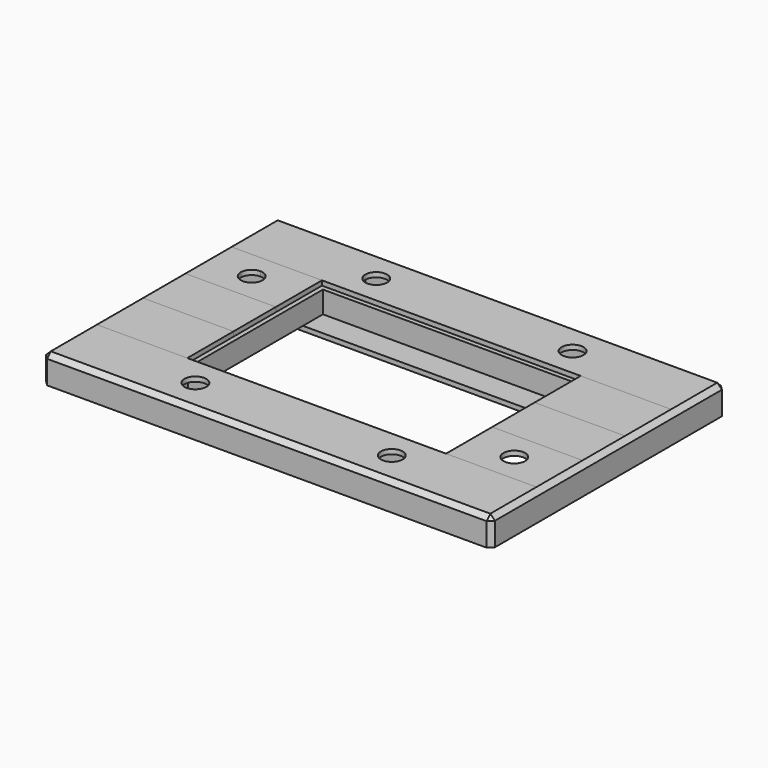
from build123d import *

# Parameters (mm, degrees)
F0_W       = 38.1
F0_H       = 38.1
F0_W_2     = 1016
F0_H_2     = 647.7
F0_W_3     = 311.15
F0_H_3     = 177.8
F1_DEPTH   = 88.9
F2_W       = 311.15
F2_H       = 177.8
F2_W_2     = 1016
F3_DEPTH   = 19.05
F2_H_2     = 215.9
F2_W_3     = 38.1
F2_W_4     = 19.05
F4_DEPTH   = 19.05
F5_W       = 1092.2
F5_H       = 139.7
F6_DEPTH   = 19.05
F7_W       = 1790.7
F7_H       = 114.3
F8_DEPTH   = 19.05
F9_W       = 1790.7
F9_H       = 114.3
F10_DEPTH  = 19.05
F11_W      = 1193.8
F11_H      = 114.3
F12_DEPTH  = 19.05
F13_W      = 1193.8
F13_H      = 114.3
F14_DEPTH  = 19.05
F15_SIZE   = 19.04999
F15_2_SIZE = 19.04999
F15_3_SIZE = 19.04999
F15_4_SIZE = 19.04999
F16_R      = 44.45
F17_DEPTH  = 19.05


# Not quite as in the source:
# - a fillet or chamfer is up to 0.001 mm smaller than in the source, because OpenCascade refuses the exact size


with BuildPart() as f1:
    # F0 (on Top) → F1 (new body)
    with BuildSketch(Plane.XY):
        with Locations((527.05, 558.8)):
            Rectangle(F0_W, F0_H)
        with Locations((0, 558.8)):
            Rectangle(F0_W_2, F0_H)
        with Locations((876.3, 0)):
            Rectangle(F0_W, F0_H_2)
        with Locations((876.3, 342.9)):
            Rectangle(F0_W, F0_H)
        with Locations((-876.3, 342.9)):
            Rectangle(F0_W, F0_H)
        with Locations((-876.3, 0)):
            Rectangle(F0_W, F0_H_2)
        with Locations((-527.05, 558.8)):
            Rectangle(F0_W, F0_H)
        with Locations((0, -558.8)):
            Rectangle(F0_W_2, F0_H)
        with Locations((527.05, -558.8)):
            Rectangle(F0_W, F0_H)
        with Locations((876.3, -342.9)):
            Rectangle(F0_W, F0_H)
        Polygon((546.1, 577.85), (546.1, 539.75), (857.25, 539.75), (857.25, 361.95), (895.35, 361.95), (895.35, 577.85), align=None)
        with Locations((-876.3, -342.9)):
            Rectangle(F0_W, F0_H)
        with Locations((-527.05, -558.8)):
            Rectangle(F0_W, F0_H)
        Polygon((-895.35, 361.95), (-857.25, 361.95), (-857.25, 539.75), (-546.1, 539.75), (-546.1, 577.85), (-895.35, 577.85), align=None)
        Polygon((857.25, -539.75), (546.1, -539.75), (546.1, -577.85), (895.35, -577.85), (895.35, -361.95), (857.25, -361.95), align=None)
        Polygon((-857.25, -539.75), (-857.25, -361.95), (-895.35, -361.95), (-895.35, -577.85), (-546.1, -577.85), (-546.1, -539.75), align=None)
        with Locations((-701.675, 342.9)):
            Rectangle(F0_W_3, F0_H)
        with Locations((-527.05, 450.85)):
            Rectangle(F0_W, F0_H_3)
        with Locations((-527.05, 342.9)):
            Rectangle(F0_W, F0_H)
        with Locations((-527.05, 0)):
            Rectangle(F0_W, F0_H_2)
        with Locations((-701.675, -342.9)):
            Rectangle(F0_W_3, F0_H)
        with Locations((-527.05, -450.85)):
            Rectangle(F0_W, F0_H_3)
        with Locations((-527.05, -342.9)):
            Rectangle(F0_W, F0_H)
        with Locations((0, -342.9)):
            Rectangle(F0_W_2, F0_H)
        with Locations((527.05, -450.85)):
            Rectangle(F0_W, F0_H_3)
        with Locations((527.05, -342.9)):
            Rectangle(F0_W, F0_H)
        with Locations((701.675, -342.9)):
            Rectangle(F0_W_3, F0_H)
        with Locations((527.05, 0)):
            Rectangle(F0_W, F0_H_2)
        with Locations((527.05, 342.9)):
            Rectangle(F0_W, F0_H)
        with Locations((527.05, 450.85)):
            Rectangle(F0_W, F0_H_3)
        with Locations((701.675, 342.9)):
            Rectangle(F0_W_3, F0_H)
        with Locations((0, 342.9)):
            Rectangle(F0_W_2, F0_H)
    extrude(amount=-F1_DEPTH)


with BuildPart() as f3:
    # F2 (on face) → F3 (new body)
    with BuildSketch(Plane.XY):
        Polygon((895.35, 577.85), (-895.35, 577.85), (-895.35, 342.9), (-527.05, 342.9), (527.05, 342.9), (895.35, 342.9), align=None)
        with Locations((-701.675, 450.85)):
            Rectangle(F2_W, F2_H, mode=Mode.SUBTRACT)
        with Locations((0, 450.85)):
            Rectangle(F2_W_2, F2_H, mode=Mode.SUBTRACT)
        with Locations((701.675, 450.85)):
            Rectangle(F2_W, F2_H, mode=Mode.SUBTRACT)
        with Locations((-701.675, 450.85)):
            Rectangle(F2_W, F2_H)
        with Locations((0, 450.85)):
            Rectangle(F2_W_2, F2_H)
        with Locations((701.675, 450.85)):
            Rectangle(F2_W, F2_H)
    extrude(amount=F3_DEPTH)


with BuildPart() as f3b:
    # F2 (on face) → F3, piece 2 (new body)
    with BuildSketch(Plane.XY):
        with Locations((701.675, 0)):
            Rectangle(F2_W, F2_H_2)
        with Locations((876.3, 0)):
            Rectangle(F2_W_3, F2_H_2)
        with Locations((536.575, 0)):
            Rectangle(F2_W_4, F2_H_2)
    extrude(amount=F3_DEPTH)


with BuildPart() as f3c:
    # F2 (on face) → F3, piece 3 (new body)
    with BuildSketch(Plane.XY):
        with Locations((-701.675, 0)):
            Rectangle(F2_W, F2_H_2)
        with Locations((-876.3, 0)):
            Rectangle(F2_W_3, F2_H_2)
        with Locations((-536.575, 0)):
            Rectangle(F2_W_4, F2_H_2)
    extrude(amount=F3_DEPTH)


with BuildPart() as f3d:
    # F2 (on face) → F3, piece 4 (new body)
    with BuildSketch(Plane.XY):
        Polygon((-527.05, -342.9), (-895.35, -342.9), (-895.35, -577.85), (895.35, -577.85), (895.35, -342.9), (527.05, -342.9), align=None)
        with Locations((-701.675, -450.85)):
            Rectangle(F2_W, F2_H, mode=Mode.SUBTRACT)
        with Locations((0, -450.85)):
            Rectangle(F2_W_2, F2_H, mode=Mode.SUBTRACT)
        with Locations((701.675, -450.85)):
            Rectangle(F2_W, F2_H, mode=Mode.SUBTRACT)
        with Locations((-701.675, -450.85)):
            Rectangle(F2_W, F2_H)
        with Locations((0, -450.85)):
            Rectangle(F2_W_2, F2_H)
        with Locations((701.675, -450.85)):
            Rectangle(F2_W, F2_H)
    extrude(amount=F3_DEPTH)


with BuildPart() as f4:
    # F2 (on face) → F4 (new body)
    with BuildSketch(Plane.XY):
        with Locations((-701.675, 215.9)):
            Rectangle(F2_W, F2_H_2)
        Polygon((-527.05, 342.9), (-895.35, 342.9), (-895.35, 107.95), (-857.25, 107.95), (-857.25, 323.85), (-546.1, 323.85), (-546.1, 107.95), (-527.05, 107.95), align=None)
    extrude(amount=F4_DEPTH)


with BuildPart() as f4b:
    # F2 (on face) → F4, piece 2 (new body)
    with BuildSketch(Plane.XY):
        Polygon((895.35, 107.95), (895.35, 342.9), (527.05, 342.9), (527.05, 107.95), (546.1, 107.95), (546.1, 323.85), (857.25, 323.85), (857.25, 107.95), align=None)
        with Locations((701.675, 215.9)):
            Rectangle(F2_W, F2_H_2)
    extrude(amount=F4_DEPTH)


with BuildPart() as f4c:
    # F2 (on face) → F4, piece 3 (new body)
    with BuildSketch(Plane.XY):
        Polygon((895.35, -342.9), (895.35, -107.95), (857.25, -107.95), (857.25, -323.85), (546.1, -323.85), (546.1, -107.95), (527.05, -107.95), (527.05, -342.9), align=None)
        with Locations((701.675, -215.9)):
            Rectangle(F2_W, F2_H_2)
    extrude(amount=F4_DEPTH)


with BuildPart() as f4d:
    # F2 (on face) → F4, piece 4 (new body)
    with BuildSketch(Plane.XY):
        Polygon((-857.25, -107.95), (-895.35, -107.95), (-895.35, -342.9), (-527.05, -342.9), (-527.05, -107.95), (-546.1, -107.95), (-546.1, -323.85), (-857.25, -323.85), align=None)
        with Locations((-701.675, -215.9)):
            Rectangle(F2_W, F2_H_2)
    extrude(amount=F4_DEPTH)


with BuildPart() as f6:
    # F5 (on face) → F6 (new body)
    with BuildSketch(Plane(origin=(0, 0, -88.9), x_dir=(1, 0, 0), z_dir=(0, 0, -1))):
        with Locations((0, 292.1)):
            Rectangle(F5_W, F5_H)
    extrude(amount=F6_DEPTH)


with BuildPart() as f6b:
    # F5 (on face) → F6, piece 2 (new body)
    with BuildSketch(Plane(origin=(0, 0, -88.9), x_dir=(1, 0, 0), z_dir=(0, 0, -1))):
        with Locations((0, -292.1)):
            Rectangle(F5_W, F5_H)
    extrude(amount=F6_DEPTH)


with BuildPart() as f8:
    # F7 (on face) → F8 (new body)
    with BuildSketch(Plane.XZ.offset(577.85)):
        with Locations((0, -38.1)):
            Rectangle(F7_W, F7_H)
    extrude(amount=F8_DEPTH)

    # F15#3 (size 19.05 in the source; OpenCascade refuses exactly that, so slightly less here)
    f15_3_edges = [f8.edges().sort_by_distance(p)[0] for p in [
        (0, -596.9, 19.05),
    ]]
    chamfer(f15_3_edges, length=F15_3_SIZE)


with BuildPart() as f10:
    # F9 (on face) → F10 (new body)
    with BuildSketch(Plane(origin=(0, 577.85, 0), x_dir=(-1, 0, 0), z_dir=(0, 1, 0))):
        with Locations((0, -38.1)):
            Rectangle(F9_W, F9_H)
    extrude(amount=F10_DEPTH)

    # F15#2 (size 19.05 in the source; OpenCascade refuses exactly that, so slightly less here)
    f15_2_edges = [f10.edges().sort_by_distance(p)[0] for p in [
        (0, 596.9, 19.05),
    ]]
    chamfer(f15_2_edges, length=F15_2_SIZE)


with BuildPart() as f12:
    # F11 (on face) → F12 (new body)
    with BuildSketch(Plane.YZ.offset(895.35)):
        with Locations((0, -38.1)):
            Rectangle(F11_W, F11_H)
    extrude(amount=F12_DEPTH)

    # F15#4 (size 19.05 in the source; OpenCascade refuses exactly that, so slightly less here)
    f15_4_edges = [f12.edges().sort_by_distance(p)[0] for p in [
        (914.4, 0, 19.05),
        (914.4, -596.9, -38.1),
        (914.4, 596.9, -38.1),
        (904.875, 596.9, 19.05),
        (904.875, -596.9, 19.05),
    ]]
    chamfer(f15_4_edges, length=F15_4_SIZE)


with BuildPart() as f14:
    # F13 (on face) → F14 (new body)
    with BuildSketch(Plane(origin=(-895.35, 0, 0), x_dir=(0, -1, 0), z_dir=(-1, 0, 0))):
        with Locations((0, -38.1)):
            Rectangle(F13_W, F13_H)
    extrude(amount=F14_DEPTH)

    # F15 (size 19.05 in the source; OpenCascade refuses exactly that, so slightly less here)
    f15_edges = [f14.edges().sort_by_distance(p)[0] for p in [
        (-914.4, 0, 19.05),
        (-914.4, 596.9, -38.1),
        (-914.4, -596.9, -38.1),
        (-904.875, -596.9, 19.05),
        (-904.875, 596.9, 19.05),
    ]]
    chamfer(f15_edges, length=F15_SIZE)


with BuildPart() as f17_tool:
    # F16 (on face) → F17 (new body)
    with BuildSketch(Plane.XY.offset(19.05)):
        with BuildLine():
            ThreePointArc((-355.6, 460.375), (-400.05, 504.825), (-444.5, 460.375))
            ThreePointArc((-444.5, 460.375), (-400.05, 415.925), (-355.6, 460.375))
        make_face()
        with Locations((400.05, 460.375)):
            Circle(F16_R)
        with BuildLine():
            ThreePointArc((755.65, -225.425), (711.2, -180.975), (666.75, -225.425))
            Line((666.75, -225.425), (755.65, -225.425))
        make_face()
        with BuildLine():
            Line((755.65, -225.425), (666.75, -225.425))
            ThreePointArc((666.75, -225.425), (711.2, -269.875), (755.65, -225.425))
        make_face()
        with Locations((400.05, -460.375)):
            Circle(F16_R)
        with BuildLine():
            ThreePointArc((-355.6, -460.375), (-400.05, -415.925), (-444.5, -460.375))
            ThreePointArc((-444.5, -460.375), (-400.05, -504.825), (-355.6, -460.375))
        make_face()
        with BuildLine():
            ThreePointArc((-719.3776369095, 180.975), (-687.9467404857, 193.9941035763), (-674.9276369095, 225.425))
            Line((-674.9276369095, 225.425), (-719.3776369095, 225.425))
            Line((-719.3776369095, 225.425), (-719.3776369095, 180.975))
        make_face()
        with BuildLine():
            Line((-719.3776369095, 225.425), (-674.9276369095, 225.425))
            ThreePointArc((-674.9276369095, 225.425), (-687.9467404857, 256.8558964237), (-719.3776369095, 269.875))
            Line((-719.3776369095, 269.875), (-719.3776369095, 225.425))
        make_face()
        with BuildLine():
            Line((-719.3776369095, 180.975), (-719.3776369095, 225.425))
            Line((-719.3776369095, 225.425), (-763.8276369095, 225.425))
            ThreePointArc((-763.8276369095, 225.425), (-750.8085333332, 193.9941035763), (-719.3776369095, 180.975))
        make_face()
        with BuildLine():
            Line((-763.8276369095, 225.425), (-719.3776369095, 225.425))
            Line((-719.3776369095, 225.425), (-719.3776369095, 269.875))
            ThreePointArc((-719.3776369095, 269.875), (-750.8085333332, 256.8558964237), (-763.8276369095, 225.425))
        make_face()
    extrude(amount=-F17_DEPTH)


with BuildPart() as f3_1:
    add(f3.part)

    # F17: cut by f17_tool
    add(f17_tool.part, mode=Mode.SUBTRACT)


with BuildPart() as f3d_1:
    add(f3d.part)

    # F17: cut by f17_tool
    add(f17_tool.part, mode=Mode.SUBTRACT)


with BuildPart() as f4_1:
    add(f4.part)

    # F17: cut by f17_tool
    add(f17_tool.part, mode=Mode.SUBTRACT)


with BuildPart() as f4c_1:
    add(f4c.part)

    # F17: cut by f17_tool
    add(f17_tool.part, mode=Mode.SUBTRACT)


solid = Compound([f1.part, f3b.part, f3c.part, f4b.part, f4d.part, f6.part, f6b.part, f8.part, f10.part, f12.part, f14.part, f3_1.part, f3d_1.part, f4_1.part, f4c_1.part])
